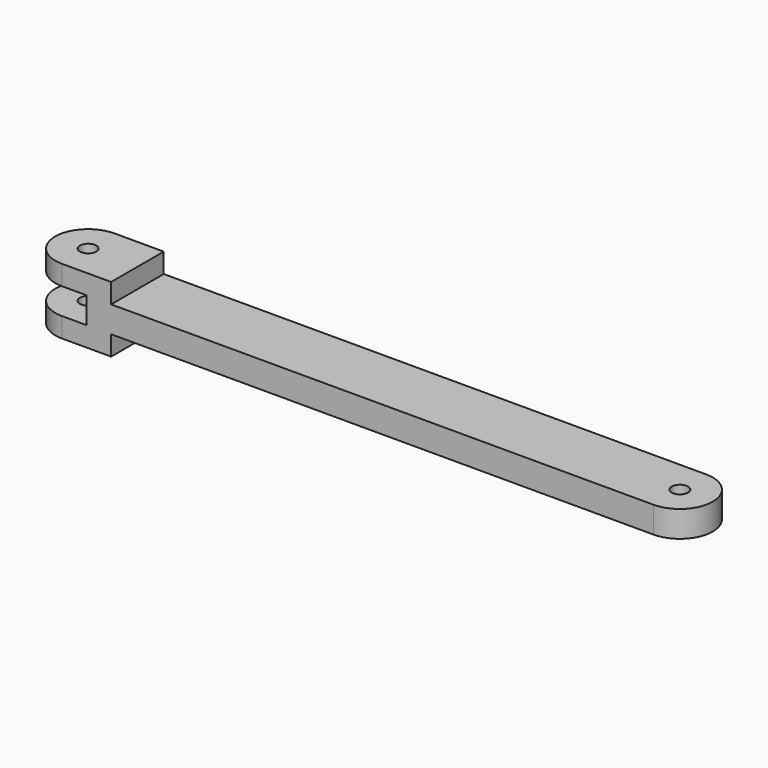
from build123d import *

# Parameters (mm, degrees)
F0_W     = 150
F0_H     = 20
F0_R     = 2.5
F1_DEPTH = 4
F2_DEPTH = 10
F3_W     = 7.5
F3_H     = 8
F3_W_2   = 10.5527898669
F4_DEPTH = 25


# Not quite as in the source:
# - a feature names something its author has since deleted; it is built from what else it names


with BuildPart() as f1:
    # F0 (on Top) → F1 (new body, symmetric)
    with BuildSketch(Plane.XY):
        Rectangle(F0_W, F0_H)
        with BuildLine():
            Line((90, 10), (75, 10))
            Line((75, 10), (75, -10))
            Line((75, -10), (90, -10))
            ThreePointArc((90, -10), (80, 0), (90, 10))
        make_face()
        with BuildLine():
            ThreePointArc((100, 0), (97.0710678119, 7.0710678119), (90, 10))
            ThreePointArc((90, 10), (80, 0), (90, -10))
            ThreePointArc((90, -10), (97.0710678119, -7.0710678119), (100, 0))
        make_face()
        with Locations((90, 0)):
            Circle(F0_R, mode=Mode.SUBTRACT)
    extrude(amount=F1_DEPTH, both=True)

    # F0 (on Top) → F2 (join, symmetric)
    with BuildSketch(Plane.XY):
        with BuildLine():
            ThreePointArc((-80, 0), (-82.9289321881, 7.0710678119), (-90, 10))
            ThreePointArc((-90, 10), (-100, 0), (-90, -10))
            ThreePointArc((-90, -10), (-82.9289321881, -7.0710678119), (-80, 0))
        make_face()
        with Locations((-90, 0)):
            Circle(F0_R, mode=Mode.SUBTRACT)
        with BuildLine():
            Line((-75, -10), (-75, 10))
            Line((-75, 10), (-90, 10))
            ThreePointArc((-90, 10), (-82.9289321881, 7.0710678119), (-80, 0))
            ThreePointArc((-80, 0), (-82.9289321881, -7.0710678119), (-90, -10))
            Line((-90, -10), (-75, -10))
        make_face()
    extrude(amount=F2_DEPTH, both=True)

    # F3 (on face) → F4 (cut)
    with BuildSketch(Plane.XZ.offset(10)):
        with Locations((-86.25, 0)):
            Rectangle(F3_W, F3_H)
        with Locations((-95.2763949335, 0)):
            Rectangle(F3_W_2, F3_H)
    extrude(amount=-F4_DEPTH, mode=Mode.SUBTRACT)


solid = f1.part
